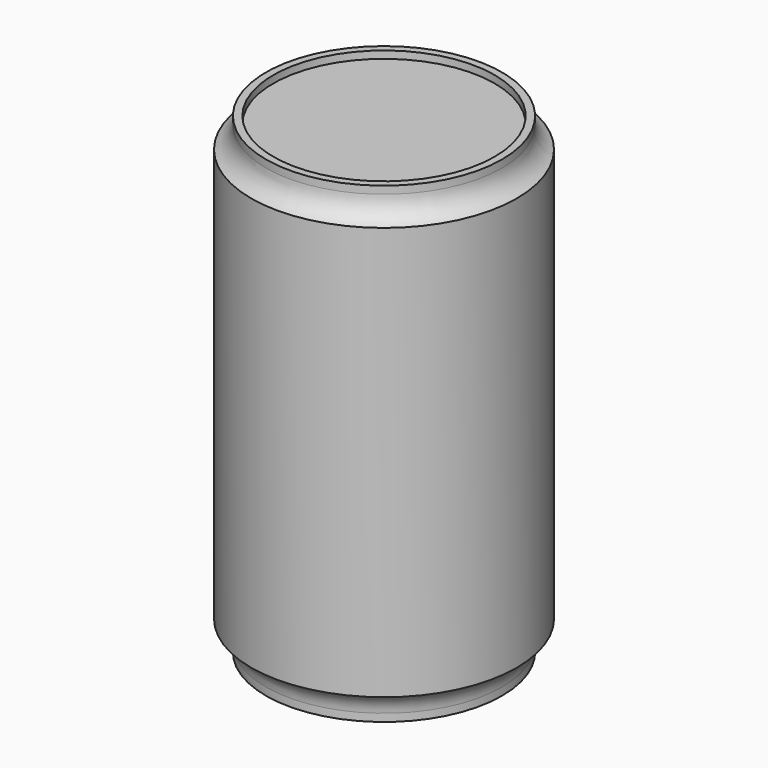
from build123d import *

# Parameters (mm, degrees)
F0_R     = 28.575
F0_R_2   = 25.4
F1_DEPTH = 95.25
F0_R_3   = 23.8125
F2_DEPTH = 101.6
F3_DEPTH = 6.35
F4_DEPTH = 100.0125
F5_DEPTH = 6.35
F6_DEPTH = 6.35
F7_R     = 5.08
F9_T     = -2.54


# Not quite as in the source:
# - a fillet or chamfer that OpenCascade refuses, or shapes differently, is made with other operations: its cross-section is extruded or revolved along the edge and cut away or added


with BuildPart() as f1:
    # F0 (on Top) → F1 (new body)
    with BuildSketch(Plane.XY):
        Circle(F0_R)
        Circle(F0_R_2, mode=Mode.SUBTRACT)
    extrude(amount=F1_DEPTH)

    # F0 (on Top) → F2 (join)
    with BuildSketch(Plane.XY):
        Circle(F0_R_2)
        Circle(F0_R_3, mode=Mode.SUBTRACT)
    extrude(amount=F2_DEPTH)

    # F0 (on Top) → F3 (cut)
    with BuildSketch(Plane.XY):
        Circle(F0_R)
        Circle(F0_R_2, mode=Mode.SUBTRACT)
    extrude(amount=F3_DEPTH, mode=Mode.SUBTRACT)

    # F0 (on Top) → F4 (join)
    with BuildSketch(Plane.XY):
        Circle(F0_R_3)
    extrude(amount=F4_DEPTH)

    # F0 (on Top) → F5 (join)
    with BuildSketch(Plane.XY):
        Circle(F0_R_3)
    extrude(amount=F5_DEPTH)

    # F0 (on Top) → F6 (cut)
    with BuildSketch(Plane.XY):
        Circle(F0_R_3)
    extrude(amount=F6_DEPTH, mode=Mode.SUBTRACT)

    # F7
    f7_edges = [f1.edges().sort_by_distance(p)[0] for p in [
        (-23.8125, 0, 6.35),
    ]]
    fillet(f7_edges, radius=F7_R)

    # F8: fillet of radius 5.08 on 2 edges, made by hand

    # F8_s1 → F8_t2 (revolve)
    with BuildSketch(Plane.XZ):
        with BuildLine():
            ThreePointArc((25.4, 1.6407139607), (26.2678865162, 4.4805202921), (28.575, 6.35))
            Line((28.575, 6.35), (25.4, 6.35))
            Line((25.4, 6.35), (25.4, 1.6407139607))
        make_face()
    revolve(axis=Axis((0, 0, 6.35), (0, 0, 1)))

    # F8_s3 → F8_t4 (revolve)
    with BuildSketch(Plane.XZ):
        with BuildLine():
            ThreePointArc((28.575, 95.25), (26.2678865162, 97.1194797079), (25.4, 99.9592860393))
            Line((25.4, 99.9592860393), (25.4, 95.25))
            Line((25.4, 95.25), (28.575, 95.25))
        make_face()
    revolve(axis=Axis((0, 0, 95.25), (0, 0, 1)))

    # F9 (hollow: no face is removed)
    offset(amount=F9_T, mode=Mode.SUBTRACT)


solid = f1.part
